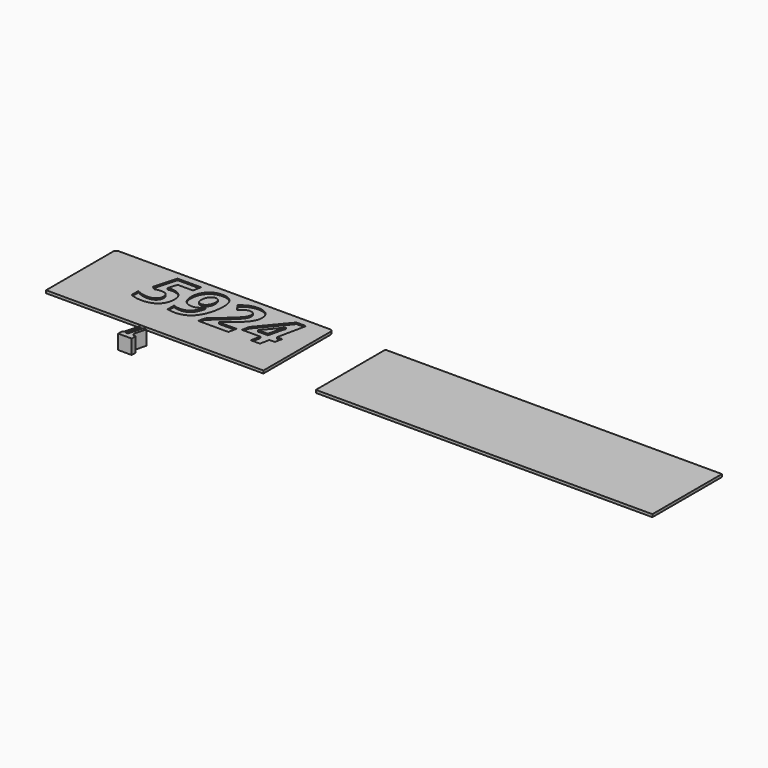
from build123d import *

# Parameters (mm, degrees)
F0_W         = 381
F0_H         = 152.4
F1_DEPTH     = 4.7625
F2_TEXT_SIZE = 112.1655934387
F3_DEPTH     = 2.5
F4_R         = 5.08
F0_W_2       = 589.9848937988
F5_DEPTH     = 4.7625
F7_DEPTH     = 25.4
F8_T1_DEPTH  = 25.4


# Not quite as in the source:
# - a fillet or chamfer that OpenCascade refuses, or shapes differently, is made with other operations: its cross-section is extruded or revolved along the edge and cut away or added
# - a length typed as a fraction of an inch, garbled in the dataset ("3 / 203.2 mm" for 3/8 in), is restored
# - Text() gives the source's letters only with a copy of the font that has no kerning and outlines rounded to 1/6400 em; it was checked with that copy


with BuildPart() as f1:
    # F0 (on Top) → F1 (new body)
    with BuildSketch(Plane.XY):
        with Locations((-15.1772722602, 82.4459424397)):
            Rectangle(F0_W, F0_H)
    extrude(amount=F1_DEPTH)

    # F2 (on face) → F3 (cut)
    with BuildSketch(Plane.XY.offset(4.7625)):
        with Locations((-107.0148286203, 65.4535144567)):
            Text('5924', F2_TEXT_SIZE, font='Open Sans', font_style=FontStyle.BOLDITALIC, text_align=(TextAlign.LEFT, TextAlign.BOTTOM))
    extrude(amount=-F3_DEPTH, mode=Mode.SUBTRACT)

    # F4
    f4_edges = [f1.edges().sort_by_distance(p)[0] for p in [
        (-205.677272, 158.645942, 2.38125),
        (175.322728, 158.645942, 2.38125),
    ]]
    fillet(f4_edges, radius=F4_R)


with BuildPart() as f5:
    # F0 (on Top) → F5 (new body)
    with BuildSketch(Plane.XY):
        with Locations((562.2366070747, 82.4459424397)):
            Rectangle(F0_W_2, F0_H)
    extrude(amount=F5_DEPTH)


with BuildPart() as f7:
    # F6 (on Top) → F7 (new body)
    with BuildSketch(Plane.XY):
        Polygon((-11.1616440852, -29.5633085206), (-14.4365432976, -29.5633085206), (-21.2424527854, -54.9633085206), (-23.3878592165, -54.9633085206), (-23.3878592165, -63.4903433365), (0.2090599215, -63.4903433365), (0.2090599215, -54.9633085206), (-7.9120192677, -54.9633085206), (-1.1061097799, -29.5633085206), (-6.3991440852, -29.5633085206), (-13.205053573, -54.9633085206), (-17.967553573, -54.9633085206), align=None)
    extrude(amount=F7_DEPTH)

    # F8: fillet of radius 5.08 on 2 edges, made by hand

    # F8_s2 → F8_t1 (join)
    with BuildSketch(Plane.XY):
        with BuildLine():
            ThreePointArc((-1.2916343736, -54.9633085206), (-5.3218693423, -52.97581658), (-6.1985375712, -48.5685077715))
            Line((-6.1985375712, -48.5685077715), (-7.9120192677, -54.9633085206))
            Line((-7.9120192677, -54.9633085206), (-1.2916343736, -54.9633085206))
        make_face()
        with BuildLine():
            ThreePointArc((-20.3265839113, -51.5452393494), (-21.4493137189, -53.6196024728), (-23.3878592165, -54.9633085206))
            Line((-23.3878592165, -54.9633085206), (-21.2424527854, -54.9633085206))
            Line((-21.2424527854, -54.9633085206), (-20.3265839113, -51.5452393494))
        make_face()
    extrude(amount=F8_T1_DEPTH)


solid = Compound([f1.part, f5.part, f7.part])
